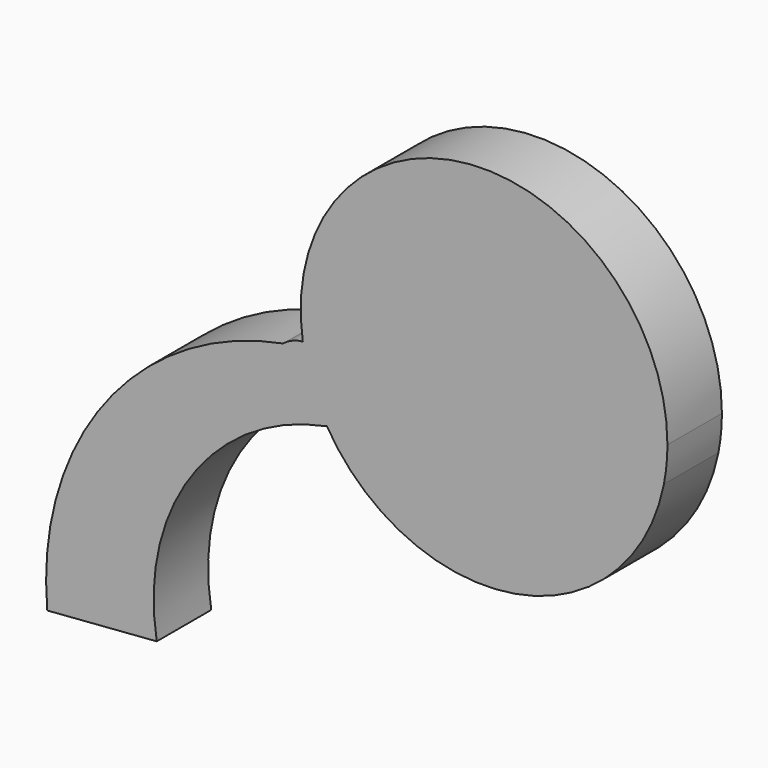
from build123d import *

# Parameters (mm, degrees)
F1_DEPTH = 7.62
F3_DEPTH = 7.62


with BuildPart() as f1:
    # F0 (on Front) → F1 (new body)
    with BuildSketch(Plane.XZ):
        with BuildLine():
            ThreePointArc((21.0290110962, 0), (21.3248501657, 1.9931047456), (21.4237811773, 4.0056155995))
            ThreePointArc((21.4237811773, 4.0056155995), (-1.1080148506, 24.4259697619), (-19.2200190896, 0))
            ThreePointArc((-19.2200190896, 0), (0.9044960033, -16.5136695746), (21.0290110962, 0))
        make_face()
    extrude(amount=F1_DEPTH)

    # F2 (on Front) → F3 (join)
    with BuildSketch(Plane.XZ):
        with BuildLine():
            ThreePointArc((-16.8698355556, -6.6087017767), (-15.6905339278, -0.7832460117), (-21.5823259205, 0))
            ThreePointArc((-21.5823259205, 0), (-41.5234625412, -12.3382675542), (-47.9722805321, -34.8836556077))
            Line((-47.9722805321, -34.8836556077), (-35.7198044658, -33.9411571622))
            ThreePointArc((-35.7198044658, -33.9411571622), (-31.8794663631, -16.423449292), (-16.8698355556, -6.6087017767))
        make_face()
    extrude(amount=F3_DEPTH)


solid = f1.part
